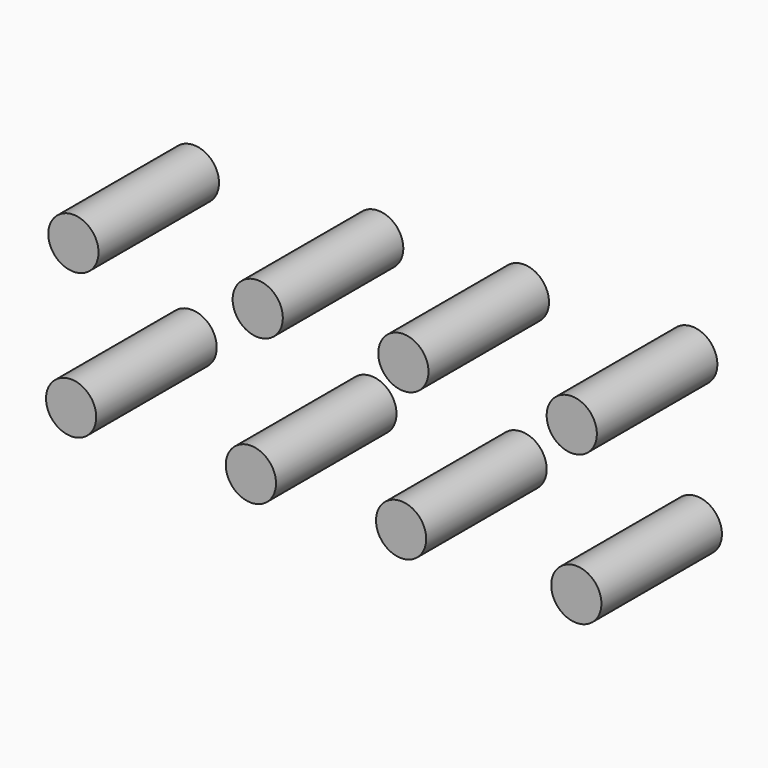
from build123d import *

# Parameters (mm, degrees)
F0_R     = 3.175
F1_DEPTH = 19.05


# Not quite as in the source:
# - a length typed as a fraction of an inch, garbled in the dataset ("3 / 203.2 mm" for 3/8 in), is restored


with BuildPart() as f1:
    # F0 (on Front) → F1 (new body)
    with BuildSketch(Plane.XZ):
        with Locations((-57.5055219233, 30.2197728306)):
            Circle(F0_R)
    extrude(amount=F1_DEPTH)


with BuildPart() as f1b:
    # F0 (on Front) → F1, piece 2 (new body)
    with BuildSketch(Plane.XZ):
        with Locations((-34.1932550073, 30.5075775832)):
            Circle(F0_R)
    extrude(amount=F1_DEPTH)


with BuildPart() as f1c:
    # F0 (on Front) → F1, piece 3 (new body)
    with BuildSketch(Plane.XZ):
        with Locations((-15.7736875117, 30.5075775832)):
            Circle(F0_R)
    extrude(amount=F1_DEPTH)


with BuildPart() as f1d:
    # F0 (on Front) → F1, piece 4 (new body)
    with BuildSketch(Plane.XZ):
        with Locations((5.5239372887, 30.5075775832)):
            Circle(F0_R)
    extrude(amount=F1_DEPTH)


with BuildPart() as f1e:
    # F0 (on Front) → F1, piece 5 (new body)
    with BuildSketch(Plane.XZ):
        with Locations((6.0995486565, 11.8002044037)):
            Circle(F0_R)
    extrude(amount=F1_DEPTH)


with BuildPart() as f1f:
    # F0 (on Front) → F1, piece 6 (new body)
    with BuildSketch(Plane.XZ):
        with Locations((-16.0614941269, 11.8002044037)):
            Circle(F0_R)
    extrude(amount=F1_DEPTH)


with BuildPart() as f1g:
    # F0 (on Front) → F1, piece 7 (new body)
    with BuildSketch(Plane.XZ):
        with Locations((-35.0566729903, 11.8002044037)):
            Circle(F0_R)
    extrude(amount=F1_DEPTH)


with BuildPart() as f1h:
    # F0 (on Front) → F1, piece 8 (new body)
    with BuildSketch(Plane.XZ):
        with Locations((-57.7933304012, 11.8002044037)):
            Circle(F0_R)
    extrude(amount=F1_DEPTH)


solid = Compound([f1.part, f1b.part, f1c.part, f1d.part, f1e.part, f1f.part, f1g.part, f1h.part])
